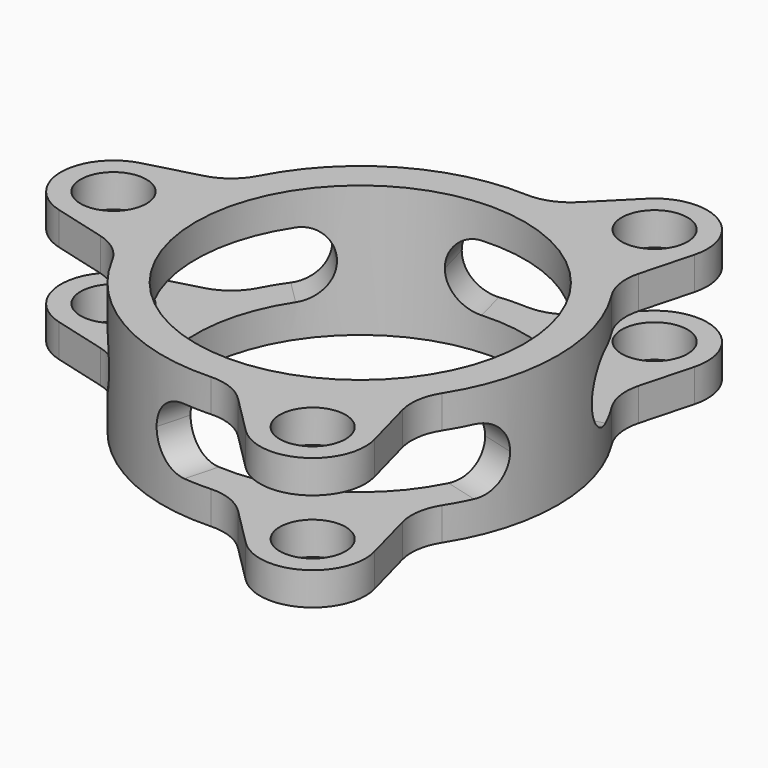
from build123d import *

# Parameters (mm, degrees)
F0_R     = 127
F0_R_2   = 635
F1_DEPTH = 254
F3_DEPTH = 127
F4_R     = 126.99999


# Not quite as in the source:
# - a fillet or chamfer is up to 0.001 mm smaller than in the source, because OpenCascade refuses the exact size


with BuildPart() as f1:
    # F0 (on Top) → F1 (new body, symmetric)
    with BuildSketch(Plane.XY):
        with BuildLine():
            ThreePointArc((-803.0204229841, -250.4210518057), (-728.5190173712, -288.1490840614), (-675.483515486, -352.6556681902))
            ThreePointArc((-675.483515486, -352.6556681902), (-381, -659.9113576837), (32.3329903017, -761.3137183436))
            ThreePointArc((32.3329903017, -761.3137183436), (381, -659.9113576837), (643.1505251843, -408.6580501534))
            ThreePointArc((643.1505251843, -408.6580501534), (762, 0), (643.1505251843, 408.6580501534))
            ThreePointArc((643.1505251843, 408.6580501534), (381, 659.9113576837), (32.3329903017, 761.3137183436))
            ThreePointArc((32.3329903017, 761.3137183436), (-381, 659.9113576837), (-675.483515486, 352.6556681902))
            ThreePointArc((-675.483515486, 352.6556681902), (-728.5190173712, 288.1490840614), (-803.0204229841, 250.4210518057))
            Line((-803.0204229841, 250.4210518057), (-1005.0920299648, 196.2761279019))
            ThreePointArc((-1005.0920299648, 196.2761279019), (-1155.7, 0), (-1005.0920299648, -196.2761279019))
            Line((-1005.0920299648, -196.2761279019), (-803.0204229841, -250.4210518057))
        make_face()
        with Locations((-952.5, 0)):
            Circle(F0_R, mode=Mode.SUBTRACT)
        Circle(F0_R_2, mode=Mode.SUBTRACT)
        with BuildLine():
            ThreePointArc((643.1505251843, -408.6580501534), (381, -659.9113576837), (32.3329903017, -761.3137183436))
            ThreePointArc((32.3329903017, -761.3137183436), (114.7150818112, -774.9905182142), (184.6392189859, -820.6466119648))
            Line((184.6392189859, -820.6466119648), (332.5659020629, -968.5732950418))
            ThreePointArc((332.5659020629, -968.5732950418), (577.85, -1000.8655591537), (672.5261279019, -772.2971671398))
            Line((672.5261279019, -772.2971671398), (618.3812039982, -570.2255601591))
            ThreePointArc((618.3812039982, -570.2255601591), (613.80393556, -486.8414341528), (643.1505251843, -408.6580501534))
        make_face()
        with Locations((476.25, -824.8891971047)):
            Circle(F0_R, mode=Mode.SUBTRACT)
        with BuildLine():
            ThreePointArc((32.3329903017, 761.3137183436), (381, 659.9113576837), (643.1505251843, 408.6580501534))
            ThreePointArc((643.1505251843, 408.6580501534), (613.80393556, 486.8414341528), (618.3812039982, 570.2255601591))
            Line((618.3812039982, 570.2255601591), (672.5261279019, 772.2971671398))
            ThreePointArc((672.5261279019, 772.2971671398), (577.85, 1000.8655591537), (332.5659020629, 968.5732950418))
            Line((332.5659020629, 968.5732950418), (184.6392189859, 820.6466119648))
            ThreePointArc((184.6392189859, 820.6466119648), (114.7150818112, 774.9905182142), (32.3329903017, 761.3137183436))
        make_face()
        with Locations((476.25, 824.8891971047)):
            Circle(F0_R, mode=Mode.SUBTRACT)
    extrude(amount=F1_DEPTH, both=True)

    # F2 (on Top) → F3 (cut, symmetric)
    with BuildSketch(Plane.XY):
        with BuildLine():
            Line((672.5261279019, -772.2971671398), (618.3812039982, -570.2255601591))
            ThreePointArc((618.3812039982, -570.2255601591), (613.80393556, -486.8414341528), (643.1505251843, -408.6580501534))
            ThreePointArc((643.1505251843, -408.6580501534), (697.6496322325, -306.4783689688), (736.0354796323, -197.2201123681))
            Line((736.0354796323, -197.2201123681), (613.3628996936, -164.3500936401))
            ThreePointArc((613.3628996936, -164.3500936401), (317.5, -549.9261314031), (-164.3500936401, -613.3628996936))
            Line((-164.3500936401, -613.3628996936), (-197.2201123681, -736.0354796323))
            ThreePointArc((-197.2201123681, -736.0354796323), (-83.4067628788, -757.4214889387), (32.3329903017, -761.3137183436))
            ThreePointArc((32.3329903017, -761.3137183436), (114.7150818112, -774.9905182142), (184.6392189859, -820.6466119648))
            Line((184.6392189859, -820.6466119648), (332.5659020629, -968.5732950418))
            ThreePointArc((332.5659020629, -968.5732950418), (577.85, -1000.8655591537), (672.5261279019, -772.2971671398))
        make_face()
        with BuildLine():
            Line((-449.0128060535, -449.0128060535), (0, 0))
            Line((0, 0), (-449.0128060535, 449.0128060535))
            ThreePointArc((-449.0128060535, 449.0128060535), (-635, 0), (-449.0128060535, -449.0128060535))
        make_face()
        with BuildLine():
            Line((-164.3500936401, 613.3628996936), (0, 0))
            Line((0, 0), (613.3628996936, 164.3500936401))
            ThreePointArc((613.3628996936, 164.3500936401), (317.5, 549.9261314031), (-164.3500936401, 613.3628996936))
        make_face()
        with BuildLine():
            ThreePointArc((-164.3500936401, -613.3628996936), (317.5, -549.9261314031), (613.3628996936, -164.3500936401))
            Line((613.3628996936, -164.3500936401), (0, 0))
            Line((0, 0), (-164.3500936401, -613.3628996936))
        make_face()
        with BuildLine():
            ThreePointArc((-449.0128060535, -449.0128060535), (-635, 0), (-449.0128060535, 449.0128060535))
            Line((-449.0128060535, 449.0128060535), (-538.8153672641, 538.8153672641))
            ThreePointArc((-538.8153672641, 538.8153672641), (-614.2428693537, 450.9431199698), (-675.483515486, 352.6556681902))
            ThreePointArc((-675.483515486, 352.6556681902), (-728.5190173712, 288.1490840614), (-803.0204229841, 250.4210518057))
            Line((-803.0204229841, 250.4210518057), (-1005.0920299648, 196.2761279019))
            ThreePointArc((-1005.0920299648, 196.2761279019), (-1155.7, 0), (-1005.0920299648, -196.2761279019))
            Line((-1005.0920299648, -196.2761279019), (-803.0204229841, -250.4210518057))
            ThreePointArc((-803.0204229841, -250.4210518057), (-728.5190173712, -288.1490840614), (-675.483515486, -352.6556681902))
            ThreePointArc((-675.483515486, -352.6556681902), (-614.2428693537, -450.9431199698), (-538.8153672641, -538.8153672641))
            Line((-538.8153672641, -538.8153672641), (-449.0128060535, -449.0128060535))
        make_face()
        with BuildLine():
            Line((-197.2201123681, 736.0354796323), (-164.3500936401, 613.3628996936))
            ThreePointArc((-164.3500936401, 613.3628996936), (317.5, 549.9261314031), (613.3628996936, 164.3500936401))
            Line((613.3628996936, 164.3500936401), (736.0354796323, 197.2201123681))
            ThreePointArc((736.0354796323, 197.2201123681), (697.6496322325, 306.4783689688), (643.1505251843, 408.6580501534))
            ThreePointArc((643.1505251843, 408.6580501534), (613.80393556, 486.8414341528), (618.3812039982, 570.2255601591))
            Line((618.3812039982, 570.2255601591), (672.5261279019, 772.2971671398))
            ThreePointArc((672.5261279019, 772.2971671398), (577.85, 1000.8655591537), (332.5659020629, 968.5732950418))
            Line((332.5659020629, 968.5732950418), (184.6392189859, 820.6466119648))
            ThreePointArc((184.6392189859, 820.6466119648), (114.7150818112, 774.9905182142), (32.3329903017, 761.3137183436))
            ThreePointArc((32.3329903017, 761.3137183436), (-83.4067628788, 757.4214889387), (-197.2201123681, 736.0354796323))
        make_face()
    extrude(amount=F3_DEPTH, both=True, mode=Mode.SUBTRACT)

    # F4 (radius 127 in the source; OpenCascade refuses exactly that, so slightly less here)
    f4_edges = [f1.edges().sort_by_distance(p)[0] for p in [
        (-180.785103, 674.69919, -127),
        (-180.785103, 674.69919, 127),
        (-493.914087, 493.914087, -127),
        (-493.914087, 493.914087, 127),
        (-493.914087, -493.914087, -127),
        (-493.914087, -493.914087, 127),
        (-180.785103, -674.69919, -127),
        (-180.785103, -674.69919, 127),
        (674.69919, -180.785103, -127),
        (674.69919, -180.785103, 127),
        (674.69919, 180.785103, -127),
        (674.69919, 180.785103, 127),
    ]]
    fillet(f4_edges, radius=F4_R)


solid = f1.part
